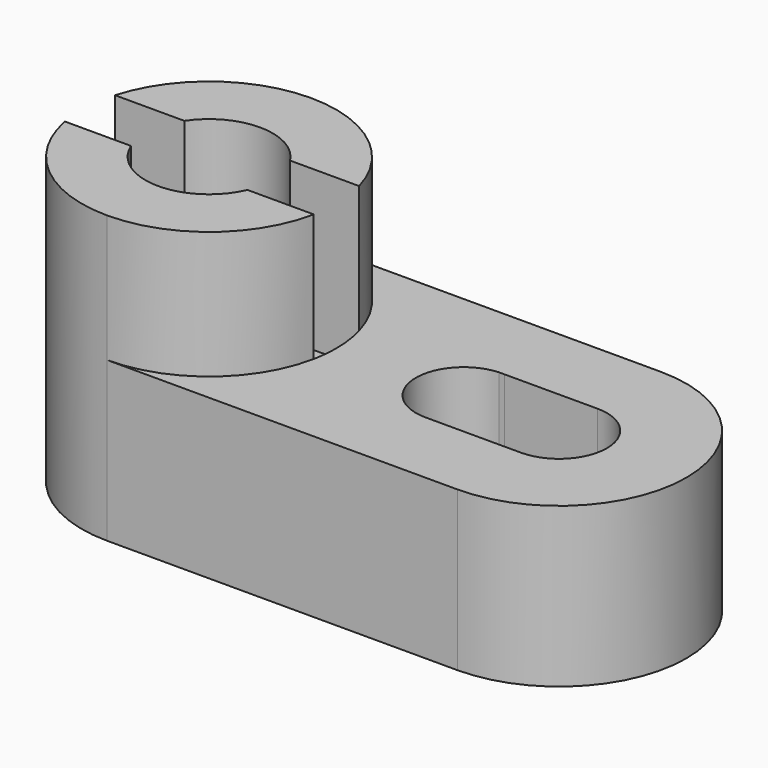
from build123d import *

# Parameters (mm, degrees)
F1_DEPTH = 25
F3_DEPTH = 20
F4_R     = 10
F5_DEPTH = 77.8
F7_DEPTH = 25
F9_DEPTH = 25


# Not quite as in the source:
# - ends of sketch curves that miss each other by under 0.0002 mm in the source are joined


with BuildPart() as f1:
    # F0 (on Top) → F1 (new body)
    with BuildSketch(Plane.XY):
        with BuildLine():
            Line((55, 20), (0, 20))
            ThreePointArc((0, 20), (-20, 0), (0, -20))
            Line((0, -20), (55, -20))
            ThreePointArc((55, -20), (75, 0), (55, 20))
        make_face()
    extrude(amount=F1_DEPTH)

    # F2 (on face) → F3 (join)
    with BuildSketch(Plane.XY.offset(25)):
        with BuildLine():
            ThreePointArc((0, -20), (14.1421356237, -14.1421356237), (20, 0))
            ThreePointArc((20, 0), (14.1421356237, 14.1421356237), (0, 20))
            ThreePointArc((0, 20), (-20, 0), (0, -20))
        make_face()
    extrude(amount=F3_DEPTH)

    # F4 (on face) → F5 (cut)
    with BuildSketch(Plane.XY.offset(45)):
        Circle(F4_R)
    extrude(amount=-F5_DEPTH, mode=Mode.SUBTRACT)

    # F6 (on face) → F7 (cut)
    with BuildSketch(Plane.XY.offset(45)):
        with BuildLine():
            ThreePointArc((-9.2726967228, -3.7439411704), (-9.9478279478, 1.02015642), (-8.3197954675, 5.5480630295))
            Line((-8.3197954675, 5.5480630295), (-19.2150721212, 5.5480630295))
            ThreePointArc((-19.2150721212, 5.5480630295), (-19.9784825468, 0.9274886135), (-19.6464476309, -3.7439411704))
            Line((-19.6464476309, -3.7439411704), (-9.2726967228, -3.7439411704))
        make_face()
        with BuildLine():
            Line((19.2537545525, 5.4122948584), (8.4087492748, 5.4122948584))
            ThreePointArc((8.4087492748, 5.4122948584), (9.593943213, 2.8206831843), (10, 0))
            ThreePointArc((10, 0), (9.7948219983, -2.0153069299), (9.1877075957, -3.94791453))
            Line((9.1877075957, -3.94791453), (19.6064777781, -3.94791453))
            ThreePointArc((19.6064777781, -3.94791453), (19.9013762786, -1.9837394534), (20, 0))
            ThreePointArc((20, 0), (19.8125602971, 2.7317493435), (19.2537545525, 5.4122948584))
        make_face()
    extrude(amount=-F7_DEPTH, mode=Mode.SUBTRACT)

    # F8 (on face) → F9 (cut)
    with BuildSketch(Plane.XY.offset(25)):
        with BuildLine():
            Line((54.9931789181, 7.4999968982), (40.4453485752, 7.4867659671))
            Line((40.4453485752, 7.4867659671), (39.5410340755, 7.485943513))
            ThreePointArc((39.5410340755, 7.485943513), (32.5035149454, -0.229590562), (40, -7.5))
            Line((40, -7.5), (55, -7.5))
            ThreePointArc((55, -7.5), (62.4999992241, 0.0034115228), (54.9931789181, 7.4999968982))
        make_face()
    extrude(amount=-F9_DEPTH, mode=Mode.SUBTRACT)


solid = f1.part
